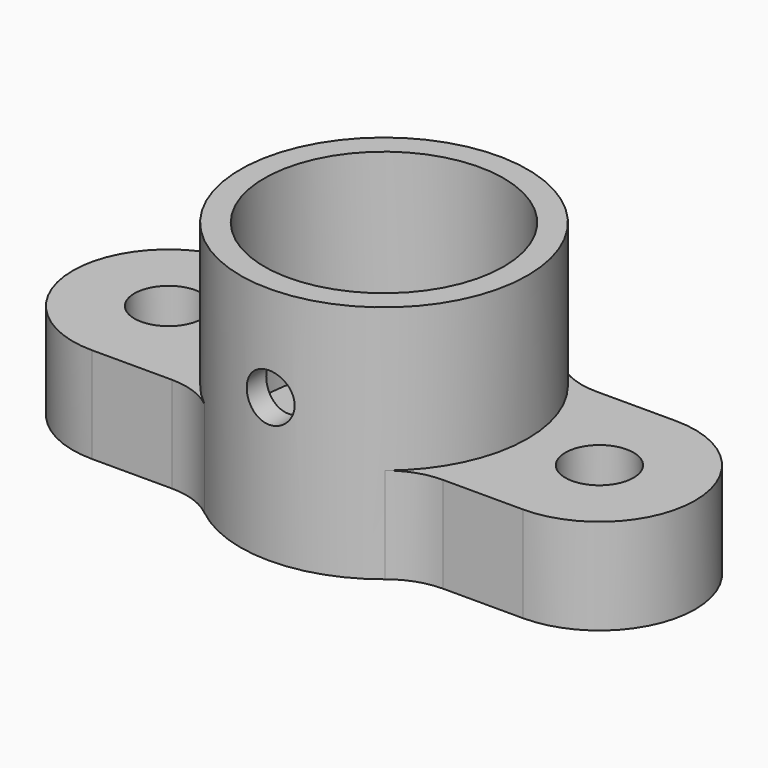
from build123d import *

# Parameters (mm, degrees)
F1_DEPTH       = 20
F2_R           = 30
F3_DEPTH       = 50
F4_R           = 25
F5_DEPTH       = 40
F7_D           = 8.8
F7_CBORE_D     = 14.25
F7_CBORE_DEPTH = 8
F8_R           = 5
F9_DEPTH       = 30.001
F10_R          = 7.5
F11_DEPTH      = 10
F12_R          = 15


# Not quite as in the source:
# - a pattern or mirror of a feature is missing from the dataset's text; its kind, count and spacing are read off the source's solid


with BuildPart() as f1:
    # F0 (on Top) → F1 (new body)
    with BuildSketch(Plane.XY):
        with BuildLine():
            Line((-45, -20), (45, -20))
            ThreePointArc((45, -20), (65, 0), (45, 20))
            Line((45, 20), (-45, 20))
            ThreePointArc((-45, 20), (-65, 0), (-45, -20))
        make_face()
    extrude(amount=F1_DEPTH)

    # F2 (on Top) → F3 (join)
    with BuildSketch(Plane.XY):
        Circle(F2_R)
    extrude(amount=F3_DEPTH)

    # F4 (on face) → F5 (cut)
    with BuildSketch(Plane.XY.offset(50)):
        Circle(F4_R)
    extrude(amount=-F5_DEPTH, mode=Mode.SUBTRACT)

    # F7 (through all)
    with Locations(Plane.XY.offset(20)):
        with Locations((45, 0)):
            f7 = CounterBoreHole(F7_D / 2, F7_CBORE_D / 2, F7_CBORE_DEPTH)

    # F7_copies: F7 across plane
    add(f7.mirror(Plane(origin=(0, 0, 0), x_dir=(0, 0, -1), z_dir=(-1, 0, 0))), mode=Mode.SUBTRACT)

    # F8 (on Front) → F9 (cut, through all)
    with BuildSketch(Plane.XZ):
        with Locations((0, 30)):
            Circle(F8_R)
    extrude(amount=F9_DEPTH, mode=Mode.SUBTRACT)

    # F10 (on face) → F11 (cut, through all)
    with BuildSketch(Plane.XY.offset(10)):
        Circle(F10_R)
    extrude(amount=-F11_DEPTH, mode=Mode.SUBTRACT)

    # F12
    f12_edges = [f1.edges().sort_by_distance(p)[0] for p in [
        (-22.36068, -20, 10),
        (22.36068, -20, 10),
        (-22.36068, 20, 10),
        (22.36068, 20, 10),
    ]]
    fillet(f12_edges, radius=F12_R)


solid = f1.part
